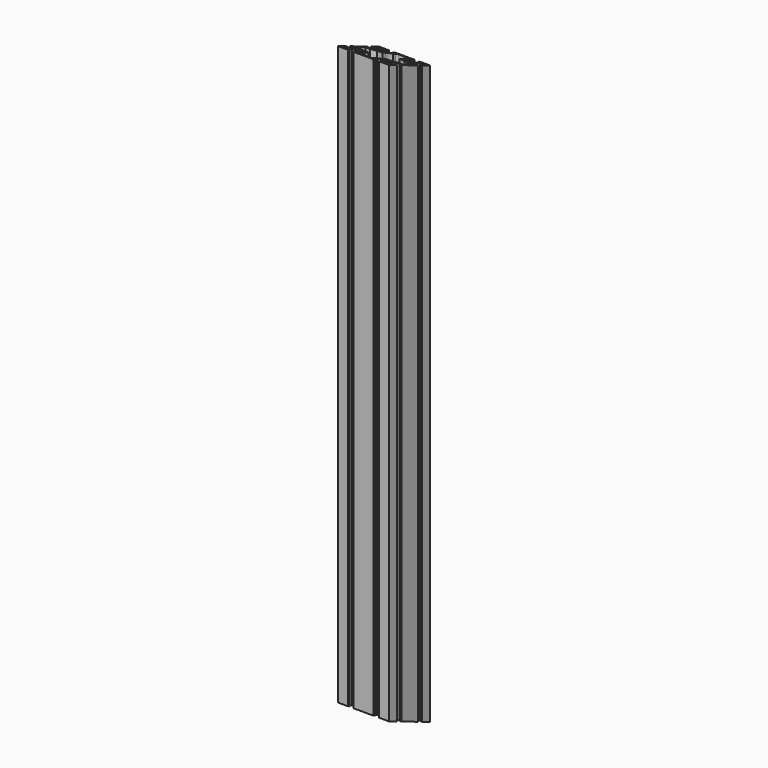
from build123d import *

# Parameters (mm, degrees)
F0_R          = 3
F0_R_2        = 2.5
F1_DEPTH      = 700
F2_R          = 2
F3_R          = 7
F6_DEPTH      = 30
F6_DEPTH_BACK = 30


# Not quite as in the source:
# - a feature names something its author has since deleted; it is built from what else it names


with BuildPart() as f1:
    # F0 (on Top) → F1 (new body)
    with BuildSketch(Plane.XY):
        with BuildLine():
            Line((18.15, -30), (30, -30))
            Line((30, -30), (30, -18.15))
            Line((30, -18.15), (27.5, -18.15))
            Line((27.5, -18.15), (27.5, -20.15))
            Line((27.5, -20.15), (21.5477069044, -20.15))
            ThreePointArc((21.5477069044, -20.15), (19.5, -15), (21.5477069044, -9.85))
            Line((21.5477069044, -9.85), (27.5, -9.85))
            Line((27.5, -9.85), (27.5, -11.85))
            Line((27.5, -11.85), (30, -11.85))
            Line((30, -11.85), (30, 11.85))
            Line((30, 11.85), (27.5, 11.85))
            Line((27.5, 11.85), (27.5, 9.85))
            Line((27.5, 9.85), (21.5477069044, 9.85))
            ThreePointArc((21.5477069044, 9.85), (19.5, 15), (21.5477069044, 20.15))
            Line((21.5477069044, 20.15), (27.5, 20.15))
            Line((27.5, 20.15), (27.5, 18.15))
            Line((27.5, 18.15), (30, 18.15))
            Line((30, 18.15), (30, 30))
            Line((30, 30), (18.15, 30))
            Line((18.15, 30), (18.15, 27.5))
            Line((18.15, 27.5), (20.15, 27.5))
            Line((20.15, 27.5), (20.15, 21.5477069044))
            ThreePointArc((20.15, 21.5477069044), (15, 19.5), (9.85, 21.5477069044))
            Line((9.85, 21.5477069044), (9.85, 27.5))
            Line((9.85, 27.5), (11.85, 27.5))
            Line((11.85, 27.5), (11.85, 30))
            Line((11.85, 30), (-11.85, 30))
            Line((-11.85, 30), (-11.85, 27.5))
            Line((-11.85, 27.5), (-9.85, 27.5))
            Line((-9.85, 27.5), (-9.85, 21.5477069044))
            ThreePointArc((-9.85, 21.5477069044), (-15, 19.5), (-20.15, 21.5477069044))
            Line((-20.15, 21.5477069044), (-20.15, 27.5))
            Line((-20.15, 27.5), (-18.15, 27.5))
            Line((-18.15, 27.5), (-18.15, 30))
            Line((-18.15, 30), (-30, 30))
            Line((-30, 30), (-30, 18.15))
            Line((-30, 18.15), (-27.5, 18.15))
            Line((-27.5, 18.15), (-27.5, 20.15))
            Line((-27.5, 20.15), (-21.5477069044, 20.15))
            ThreePointArc((-21.5477069044, 20.15), (-19.5, 15), (-21.5477069044, 9.85))
            Line((-21.5477069044, 9.85), (-27.5, 9.85))
            Line((-27.5, 9.85), (-27.5, 11.85))
            Line((-27.5, 11.85), (-30, 11.85))
            Line((-30, 11.85), (-30, -11.85))
            Line((-30, -11.85), (-27.5, -11.85))
            Line((-27.5, -11.85), (-27.5, -9.85))
            Line((-27.5, -9.85), (-21.5477069044, -9.85))
            ThreePointArc((-21.5477069044, -9.85), (-19.5, -15), (-21.5477069044, -20.15))
            Line((-21.5477069044, -20.15), (-27.5, -20.15))
            Line((-27.5, -20.15), (-27.5, -18.15))
            Line((-27.5, -18.15), (-30, -18.15))
            Line((-30, -18.15), (-30, -30))
            Line((-30, -30), (-18.15, -30))
            Line((-18.15, -30), (-18.15, -27.5))
            Line((-18.15, -27.5), (-20.15, -27.5))
            Line((-20.15, -27.5), (-20.15, -21.5477069044))
            ThreePointArc((-20.15, -21.5477069044), (-15, -19.5), (-9.85, -21.5477069044))
            Line((-9.85, -21.5477069044), (-9.85, -27.5))
            Line((-9.85, -27.5), (-11.85, -27.5))
            Line((-11.85, -27.5), (-11.85, -30))
            Line((-11.85, -30), (11.85, -30))
            Line((11.85, -30), (11.85, -27.5))
            Line((11.85, -27.5), (9.85, -27.5))
            Line((9.85, -27.5), (9.85, -21.5477069044))
            ThreePointArc((9.85, -21.5477069044), (15, -19.5), (20.15, -21.5477069044))
            Line((20.15, -21.5477069044), (20.15, -27.5))
            Line((20.15, -27.5), (18.15, -27.5))
            Line((18.15, -27.5), (18.15, -30))
        make_face()
        with Locations((-25, -25)):
            Circle(F0_R, mode=Mode.SUBTRACT)
        with Locations((-15, -15)):
            Circle(F0_R_2, mode=Mode.SUBTRACT)
        with Locations((25, -25)):
            Circle(F0_R, mode=Mode.SUBTRACT)
        with Locations((15, -15)):
            Circle(F0_R_2, mode=Mode.SUBTRACT)
        with Locations((-25, 25)):
            Circle(F0_R, mode=Mode.SUBTRACT)
        with Locations((-15, 15)):
            Circle(F0_R_2, mode=Mode.SUBTRACT)
        Polygon((-7, 22), (-7, 27.5), (0, 27.5), (7, 27.5), (7, 22), (10, 16), (10, 10), (16, 10), (22, 7), (27.5, 7), (27.5, 0), (27.5, -7), (22, -7), (16, -10), (10, -10), (10, -16), (7, -22), (7, -27.5), (0, -27.5), (-7, -27.5), (-7, -22), (-10, -16), (-10, -10), (-16, -10), (-22, -7), (-27.5, -7), (-27.5, 0), (-27.5, 7), (-22, 7), (-16, 10), (-10, 10), (-10, 16), align=None, mode=Mode.SUBTRACT)
        with Locations((15, 15)):
            Circle(F0_R_2, mode=Mode.SUBTRACT)
        with Locations((25, 25)):
            Circle(F0_R, mode=Mode.SUBTRACT)
    extrude(amount=F1_DEPTH)

    # F2
    f2_edges = [f1.edges().sort_by_distance(p)[0] for p in [
        (-7, 27.5, 350),
        (7, 27.5, 350),
    ]]
    fillet(f2_edges, radius=F2_R)

    # F3
    f3_edges = [f1.edges().sort_by_distance(p)[0] for p in [
        (-10, 16, 350),
        (10, 16, 350),
    ]]
    fillet(f3_edges, radius=F3_R)

    # F5 (on Right) → F6 (cut, two sides)
    with BuildSketch(Plane.YZ) as f6_sk:
        Polygon((30, 0), (-73.1568263622, 42.7289565306), (-138.818297568, -115.7918577799), (-35.6614712058, -158.5208143105), align=None)
        Polygon((194.2250905883, 866.574744896), (61.7300701058, 921.4559793268), (-30, 700), (102.4950204826, 645.1187655692), align=None)
    extrude(amount=F6_DEPTH, mode=Mode.SUBTRACT)
    extrude(f6_sk.sketch, amount=-F6_DEPTH_BACK, mode=Mode.SUBTRACT)


solid = f1.part
